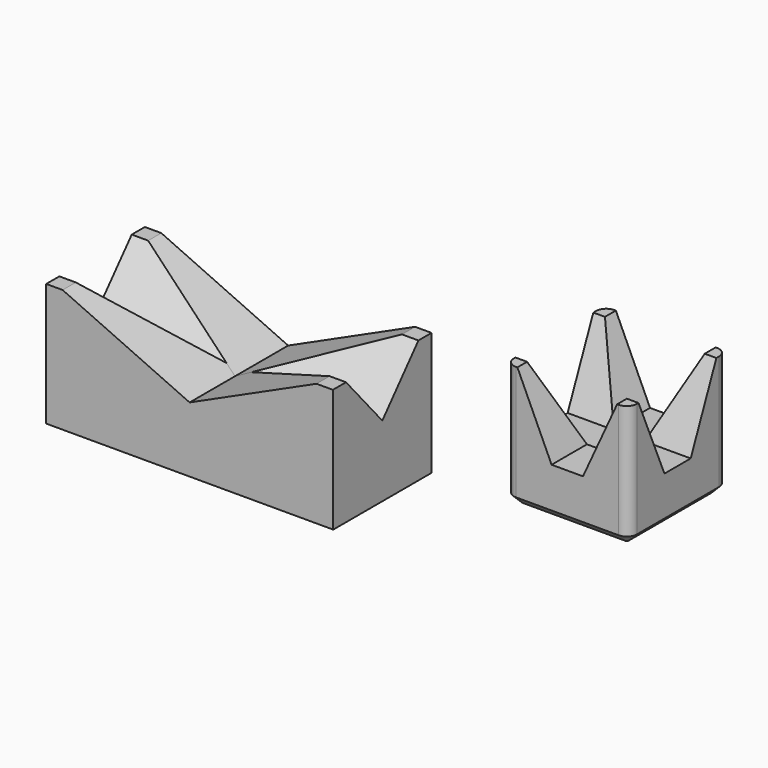
from build123d import *

# Parameters (mm, degrees)
F0_W      = 70
F0_H      = 30
F2_W      = 4
F2_H      = 4
F7_W      = 30
F7_H      = 30
F8_DEPTH  = 30
F10_DEPTH = 30
F12_DEPTH = 30
F13_R     = 2.5
F14_SIZE  = 2
F16_DEPTH = 1


# Not quite as in the source:
# - the program builds the solid bodies; features that only make, move or delete a surface that nothing else refers to are left out


with BuildPart() as f3:
    # F0 (on Top) → F3 section 0
    with BuildSketch(Plane.XY):
        Rectangle(F0_W, F0_H)
    # F2 (on offset) → F3 section 1
    with BuildSketch(Plane.XY.offset(30)):
        with Locations((-32.9428877234, 13.0318499655)):
            Rectangle(F2_W, F2_H)
    loft()

    # F0 (on Top) → F4 section 0
    with BuildSketch(Plane.XY):
        Rectangle(F0_W, F0_H)
    # F2 (on offset) → F4 section 1
    with BuildSketch(Plane.XY.offset(30)):
        with Locations((-32.9428877234, -13.0318499655)):
            Rectangle(F2_W, F2_H)
    loft()

    # F0 (on Top) → F5 section 0
    with BuildSketch(Plane.XY):
        Rectangle(F0_W, F0_H)
    # F2 (on offset) → F5 section 1
    with BuildSketch(Plane.XY.offset(30)):
        with Locations((32.9428877234, 13.0318499655)):
            Rectangle(F2_W, F2_H)
    loft()

    # F0 (on Top) → F6 section 0
    with BuildSketch(Plane.XY):
        Rectangle(F0_W, F0_H)
    # F2 (on offset) → F6 section 1
    with BuildSketch(Plane.XY.offset(30)):
        with Locations((32.9428877234, -13.0318499655)):
            Rectangle(F2_W, F2_H)
    loft()

    # F15 (on face) → F16 (cut)
    with BuildSketch(Plane.XY):
        with BuildLine():
            Line((35.1080348898, -15.1526350975), (34.9516024797, -15.1445783328))
            add(Edge.make_bspline(
                [(34.9516024797, -15.1445783328), (35.015165041, -15.1823826041), (35.0943421483, -15.2143125307), (35.1068899686, -15.1744342874), (35.1080348898, -15.1526350975)],
                knots=[0.9766966093, 0.9766966093, 0.9766966093, 0.9766966093, 0.9875020446, 0.9956975312, 0.9956975312, 0.9956975312, 0.9956975312], degree=3))
        make_face()
        with BuildLine():
            add(Edge.make_bspline(
                [(34.9719375372, 15.0837432593), (34.3538024078, 14.0181605259), (33.061090265, 11.7896967595), (28.21171153, 13.2006080373), (27.1952390941, 9.3934277248), (29.922433417, 8.7236693731), (30.66603681, 5.9963298393), (28.2491739951, 4.334922985), (27.3280801702, 1.5528957375), (30.0258958231, -0.6289713137), (28.5607968581, -2.7152455487), (26.9189490059, -6.683113184), (28.0022887063, -10.124238159), (31.4043979295, -12.0624753884), (34.4968064554, -14.8740852642), (34.9516024797, -15.1445783328)],
                knots=[0, 0, 0, 0, 0.0798778427, 0.1670493267, 0.2351952706, 0.3009592707, 0.365159693, 0.4364229102, 0.5052200474, 0.5772019582, 0.6402928372, 0.7295168151, 0.8063783849, 0.8993827171, 0.9766966093, 0.9766966093, 0.9766966093, 0.9766966093], degree=3))
            Line((34.9719375372, 15.0837432593), (30.7977404445, 15.1190953329))
            add(Edge.make_bspline(
                [(30.7977404445, 15.1190953329), (27.9337164263, 14.9101728987), (23.2612948103, 14.5693329856), (21.9160397808, 10.5126541312), (24.7378669193, 8.603835829), (26.4017007473, 6.8089006332), (24.7706534907, 4.1161935184), (23.430847623, 2.0997794876), (24.2510655844, -0.0048017343), (23.8127653987, -3.4550826329), (22.7751457805, -5.8090586344), (23.1402314335, -9.1926239549), (26.1749460731, -14.6137627403), (29.3308994565, -14.8300937762), (30.7977404445, -14.9306412786)],
                knots=[0, 0, 0, 0, 0.1234279581, 0.2013626477, 0.2811427777, 0.3472159084, 0.4234693912, 0.4927276654, 0.5582341134, 0.6420069112, 0.7141429329, 0.7966122672, 0.9054683556, 1, 1, 1, 1], degree=3))
            Line((30.7977404445, -14.9306412786), (34.9516024797, -15.1445783328))
        make_face()
        with BuildLine():
            Line((-30.7977404445, 15.1190953329), (-34.9719375372, 15.0837432593))
            add(Edge.make_bspline(
                [(-34.9719375372, 15.0837432593), (-34.3538024078, 14.0181605259), (-33.061090265, 11.7896967595), (-28.21171153, 13.2006080373), (-27.1952390941, 9.3934277248), (-29.922433417, 8.7236693731), (-30.66603681, 5.9963298393), (-28.2491739951, 4.334922985), (-27.3280801702, 1.5528957375), (-30.0258958231, -0.6289713137), (-28.5607968581, -2.7152455487), (-26.9189490059, -6.683113184), (-28.0022887063, -10.124238159), (-31.5081547913, -12.1215873684), (-34.7720178817, -15.125865809), (-35.0565479429, -15.1937999645)],
                knots=[0, 0, 0, 0, 0.0798778427, 0.1670493267, 0.2351952706, 0.3009592707, 0.365159693, 0.4364229102, 0.5052200474, 0.5772019582, 0.6402928372, 0.7295168151, 0.8063783849, 0.8993827171, 0.9842350503, 0.9842350503, 0.9842350503, 0.9842350503], degree=3))
            Line((-35.0565479429, -15.1937999645), (-30.7977404445, -14.9306412786))
            add(Edge.make_bspline(
                [(-30.7977404445, 15.1190953329), (-27.9337164263, 14.9101728987), (-23.2612948103, 14.5693329856), (-21.9160397808, 10.5126541312), (-24.7378669193, 8.603835829), (-26.4017007473, 6.8089006332), (-24.7706534907, 4.1161935184), (-23.430847623, 2.0997794876), (-24.2510655844, -0.0048017343), (-23.8127653987, -3.4550826329), (-22.7751457805, -5.8090586344), (-23.1402314335, -9.1926239549), (-26.1749460731, -14.6137627403), (-29.3308994565, -14.8300937762), (-30.7977404445, -14.9306412786)],
                knots=[0, 0, 0, 0, 0.1234279581, 0.2013626477, 0.2811427777, 0.3472159084, 0.4234693912, 0.4927276654, 0.5582341134, 0.6420069112, 0.7141429329, 0.7966122672, 0.9054683556, 1, 1, 1, 1], degree=3))
        make_face()
        with BuildLine():
            add(Edge.make_bspline(
                [(-35.0565479429, -15.1937999645), (-35.067502952, -15.1964155731), (-35.0765714389, -15.197007162), (-35.0836701691, -15.1954758912)],
                knots=[0.9842350503, 0.9842350503, 0.9842350503, 0.9842350503, 0.9875020446, 0.9875020446, 0.9875020446, 0.9875020446], degree=3))
            Line((-35.0565479429, -15.1937999645), (-35.0836701691, -15.1954758912))
        make_face()
    extrude(amount=-F16_DEPTH, mode=Mode.SUBTRACT)


with BuildPart() as f8:
    # F7 (on Top) → F8 (new body)
    with BuildSketch(Plane.XY):
        with Locations((68.754363209, 29.132604003)):
            Rectangle(F7_W, F7_H)
    extrude(amount=F8_DEPTH)

    # F9 (on face) → F10 (cut)
    with BuildSketch(Plane.XZ.offset(-14.132604003)):
        Polygon((80.9148873389, 30), (56.5938390791, 30), (64.9274835954, 11.818955776), (68.754363209, 11.818955776), (72.5812428226, 11.818955776), align=None)
    extrude(amount=-F10_DEPTH, mode=Mode.SUBTRACT)

    # F11 (on face) → F12 (cut)
    with BuildSketch(Plane.YZ.offset(83.754363209)):
        Polygon((40.8168919384, 30), (17.0854497701, 30), (24.9892928991, 11.6280304868), (32.9892928991, 11.6280304868), align=None)
    extrude(amount=-F12_DEPTH, mode=Mode.SUBTRACT)

    # F13
    f13_edges = [f8.edges().sort_by_distance(p)[0] for p in [
        (83.754363, 14.132604, 15),
        (53.754363, 14.132604, 15),
        (83.754363, 44.132604, 15),
        (53.754363, 44.132604, 15),
    ]]
    fillet(f13_edges, radius=F13_R)

    # F14
    f14_edges = [f8.edges().sort_by_distance(p)[0] for p in [
        (83.754363, 29.132604, 0),
    ]]
    chamfer(f14_edges, length=F14_SIZE)


solid = Compound([f3.part, f8.part])
